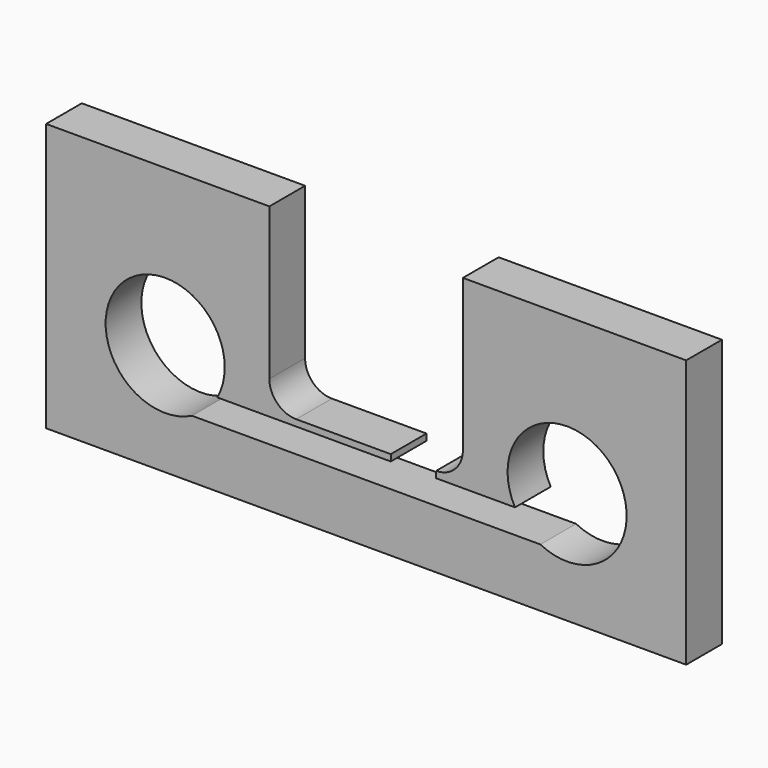
from build123d import *

# Parameters (mm, degrees)
F0_W     = 273.05
F0_H     = 114.3
F1_DEPTH = 19.05
F2_R     = 25.4
F3_DEPTH = 25.4
F5_DEPTH = 25.4
F7_DEPTH = 25.4
F8_W     = 19.3382904482
F8_H     = 2.7599734166
F9_DEPTH = 25.4


# Not quite as in the source:
# - a feature names something its author has since deleted; it is built from what else it names


with BuildPart() as f1:
    # F0 (on Front) → F1 (new body)
    with BuildSketch(Plane.XZ):
        with Locations((136.525, 57.15)):
            Rectangle(F0_W, F0_H)
    extrude(amount=F1_DEPTH)

    # F2 (on face) → F3 (cut)
    with BuildSketch(Plane.XZ.offset(19.05)):
        with Locations((50.8, 47.625)):
            Circle(F2_R)
        with Locations((222.25, 47.625)):
            Circle(F2_R)
    extrude(amount=-F3_DEPTH, mode=Mode.SUBTRACT)

    # F4 (on face) → F5 (cut)
    with BuildSketch(Plane.XZ.offset(19.05)):
        with BuildLine():
            Line((200.0185036906, 35.3400265834), (73.0314963094, 35.3400265834))
            ThreePointArc((73.0314963094, 35.3400265834), (68.4136636998, 29.3242117364), (62.225616864, 24.9398665581))
            Line((62.225616864, 24.9398665581), (210.824383136, 24.9398665581))
            ThreePointArc((210.824383136, 24.9398665581), (204.6363363002, 29.3242117364), (200.0185036906, 35.3400265834))
        make_face()
    extrude(amount=-F5_DEPTH, mode=Mode.SUBTRACT)

    # F6 (on face) → F7 (cut)
    with BuildSketch(Plane.XZ.offset(19.05)):
        with BuildLine():
            Line((177.8, 114.3), (95.25, 114.3))
            Line((95.25, 114.3), (95.25, 49.53))
            ThreePointArc((95.25, 49.53), (98.597769491, 41.447769491), (106.68, 38.1))
            Line((106.68, 38.1), (166.37, 38.1))
            ThreePointArc((166.37, 38.1), (174.452230509, 41.447769491), (177.8, 49.53))
            Line((177.8, 49.53), (177.8, 114.3))
        make_face()
    extrude(amount=-F7_DEPTH, mode=Mode.SUBTRACT)

    # F8 (on face) → F9 (cut)
    with BuildSketch(Plane.XZ.offset(19.05)):
        with Locations((156.7008547759, 36.7200132917)):
            Rectangle(F8_W, F8_H)
    extrude(amount=-F9_DEPTH, mode=Mode.SUBTRACT)


solid = f1.part
